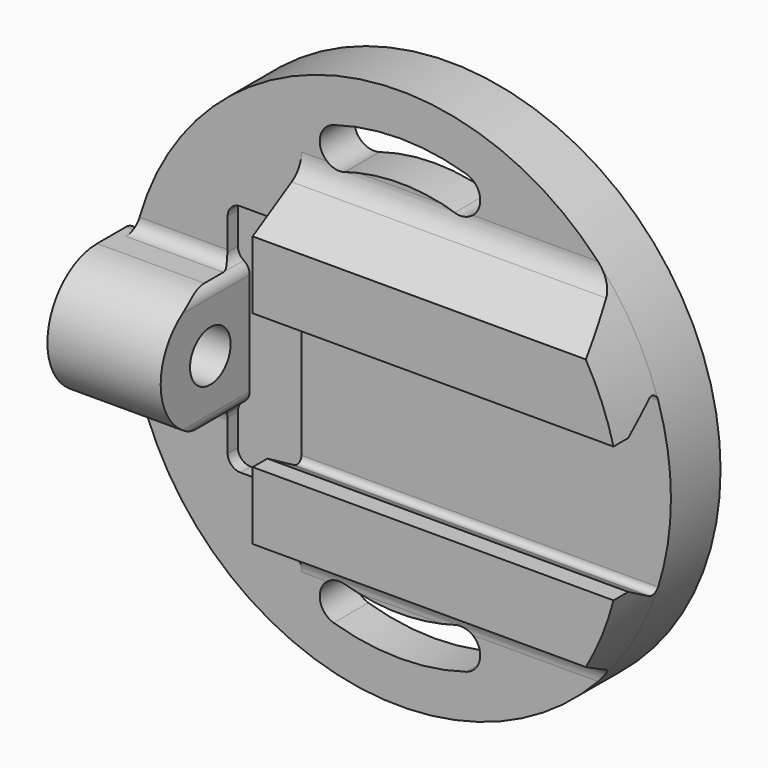
from build123d import *

# Parameters (mm, degrees)
F0_R           = 5.5025
F1_DEPTH       = 1.26
F2_R           = 5.03
F3_DEPTH       = 0.38
F4_R           = 2.75
F5_DEPTH       = 0.26
F7_DEPTH       = 7.5
F9_DEPTH       = 0.26
F10_R          = 0.26
F13_DEPTH      = 2.3
F14_R          = 0.765
F15_DEPTH      = 0.38
F16_R          = 0.515
F17_DEPTH      = 10.6835
F18_DEPTH      = 1.5
F19_F1_R       = 0.26
F19_F2_R       = 0.26
F21_DEPTH      = 15
F23_END_RADIUS = 5.5025
F23_REACH      = 10.1867902517
F25_DEPTH      = 10


# Not quite as in the source:
# - after a boolean that leaves OpenCascade's solid faulty, fix() repairs it


with BuildPart() as f1:
    # F0 (on Front) → F1 (new body)
    with BuildSketch(Plane.XZ):
        Circle(F0_R)
    extrude(amount=F1_DEPTH)

    # F2 (on face) → F3 (cut)
    with BuildSketch(Plane(origin=(0, 0, 0), x_dir=(-1, 0, 0), z_dir=(0, 1, 0))):
        Circle(F2_R)
    extrude(amount=-F3_DEPTH, mode=Mode.SUBTRACT)

    # F4 (on face) → F5 (cut)
    with BuildSketch(Plane(origin=(0, -0.38, 0), x_dir=(-1, 0, 0), z_dir=(0, 1, 0))):
        Circle(F4_R)
    extrude(amount=-F5_DEPTH, mode=Mode.SUBTRACT)

    # F6 (on face) → F7 (cut, symmetric)
    with BuildSketch(Plane.XZ.offset(1.26)):
        with BuildLine():
            ThreePointArc((-1.1142352941, 3.6852380804), (0, 3.85), (1.1142352941, 3.6852380804))
            ThreePointArc((1.1142352941, 3.6852380804), (1.6128818785, 3.952355253), (1.3457647059, 4.4510018374))
            ThreePointArc((1.3457647059, 4.4510018374), (0, 4.65), (-1.3457647059, 4.4510018374))
            ThreePointArc((-1.3457647059, 4.4510018374), (-1.6128818785, 3.952355253), (-1.1142352941, 3.6852380804))
        make_face()
        with BuildLine():
            ThreePointArc((1.1142352941, -3.6852380804), (0, -3.85), (-1.1142352941, -3.6852380804))
            ThreePointArc((-1.1142352941, -3.6852380804), (-1.6128818785, -3.952355253), (-1.3457647059, -4.4510018374))
            ThreePointArc((-1.3457647059, -4.4510018374), (0, -4.65), (1.3457647059, -4.4510018374))
            ThreePointArc((1.3457647059, -4.4510018374), (1.6128818785, -3.952355253), (1.1142352941, -3.6852380804))
        make_face()
    extrude(amount=F7_DEPTH, both=True, mode=Mode.SUBTRACT)

    # F8 (on face) → F9 (cut)
    with BuildSketch(Plane.XZ.offset(1.26)):
        with BuildLine():
            Line((-2, -2.38), (-2, 2.38))
            Line((-2, 2.38), (-3.5, 2.38))
            Line((-3.5, 2.38), (-3.5, 1.479089023))
            ThreePointArc((-3.5, 1.479089023), (-3.468035085, 1.354189063), (-3.38, 1.26))
            ThreePointArc((-3.38, 1.26), (-3.291964915, 1.165810937), (-3.26, 1.040910977))
            Line((-3.26, 1.040910977), (-3.26, -1.040910977))
            ThreePointArc((-3.26, -1.040910977), (-3.291964915, -1.165810937), (-3.38, -1.26))
            ThreePointArc((-3.38, -1.26), (-3.468035085, -1.354189063), (-3.5, -1.479089023))
            Line((-3.5, -1.479089023), (-3.5, -2.38))
            Line((-3.5, -2.38), (-2, -2.38))
        make_face()
    extrude(amount=-F9_DEPTH, mode=Mode.SUBTRACT)

    # F10
    f10_edges = [f1.edges().sort_by_distance(p)[0] for p in [
        (-2, -1.13, 2.38),
        (-3.5, -1.13, 2.38),
        (-3.5, -1.13, -2.38),
        (-2, -1.13, -2.38),
    ]]
    fillet(f10_edges, radius=F10_R)

    # F12 (on offset) → F13 (join, through all)
    with BuildSketch(Plane.YZ.offset(-5.56)):
        with BuildLine():
            Line((-1, -1.26), (-1, 1.26))
            Line((-1, 1.26), (-2, 1.26))
            ThreePointArc((-2, 1.26), (-3.26, 0), (-2, -1.26))
            Line((-2, -1.26), (-1, -1.26))
        make_face()
    extrude(amount=F13_DEPTH)

    # F14 (on face) → F15 (cut)
    with BuildSketch(Plane(origin=(-5.56, 0, 0), x_dir=(0, -1, 0), z_dir=(-1, 0, 0))):
        with Locations((2, 0)):
            Circle(F14_R)
    extrude(amount=-F15_DEPTH, mode=Mode.SUBTRACT)

    # F16 (on face) → F17 (cut, through all)
    with BuildSketch(Plane(origin=(-5.18, 0, 0), x_dir=(0, -1, 0), z_dir=(-1, 0, 0))):
        with Locations((2, 0)):
            Circle(F16_R)
    extrude(amount=-F17_DEPTH, mode=Mode.SUBTRACT)

    # F18 (cut): a face of the model
    f18_faces = [f1.faces().sort_by_distance(p)[0] for p in [
        (-2.6893148123, -1, 0),
    ]]
    extrude(f18_faces, amount=F18_DEPTH, mode=Mode.SUBTRACT)

    # F19: fillet of radius 0.26 on 4 edges, made by hand

    # F19_f1
    f19_f1_edges = [f1.edges().sort_by_distance(p)[0] for p in [
        (-5.4581479725, -1, 1.26),
        (-5.4581479725, -1, -1.26),
    ]]
    fillet(f19_f1_edges, radius=F19_F1_R)

    # F19_f2
    f19_f2_edges = [f1.edges().sort_by_distance(p)[0] for p in [
        (-4.3681479725, -1.26, 1.26),
        (-4.3681479725, -1.26, -1.26),
    ]]
    fillet(f19_f2_edges, radius=F19_F2_R)

    # F20 (on face) → F21 (cut)
    with BuildSketch(Plane.XZ.offset(1)):
        with BuildLine():
            ThreePointArc((-2.26, -2.38), (-2.0761522369, -2.3038477631), (-2, -2.12))
            Line((-2, -2.12), (-2, 2.12))
            ThreePointArc((-2, 2.12), (-2.0761522369, 2.3038477631), (-2.26, 2.38))
            Line((-2.26, 2.38), (-3.24, 2.38))
            ThreePointArc((-3.24, 2.38), (-3.4238477631, 2.3038477631), (-3.5, 2.12))
            Line((-3.5, 2.12), (-3.5, 1.479089023))
            ThreePointArc((-3.5, 1.479089023), (-3.468035085, 1.354189063), (-3.38, 1.26))
            ThreePointArc((-3.38, 1.26), (-3.2919649151, 1.165810937), (-3.2600000001, 1.0409109771))
            Line((-3.2600000001, 1.0409109771), (-3.2599999999, -1.0409109769))
            ThreePointArc((-3.2599999999, -1.0409109769), (-3.2919649149, -1.1658109369), (-3.38, -1.26))
            ThreePointArc((-3.38, -1.26), (-3.468035085, -1.354189063), (-3.5, -1.479089023))
            Line((-3.5, -1.479089023), (-3.5, -2.12))
            ThreePointArc((-3.5, -2.12), (-3.4238477631, -2.3038477631), (-3.24, -2.38))
            Line((-3.24, -2.38), (-2.26, -2.38))
        make_face()
    extrude(amount=F21_DEPTH, mode=Mode.SUBTRACT)

    f23_end = (Plane.ZX.offset(-0.76) * Cylinder(F23_END_RADIUS, 52.2556470224, mode=Mode.PRIVATE)).faces().sort_by_distance((-5.5025, -0.76, 0))[0]
    # F22 (on face) → F23 (join, up to the whole of a round face its end follows)
    with BuildSketch(Plane(origin=(-2, 0, 0), x_dir=(0, -1, 0), z_dir=(-1, 0, 0))):
        with BuildLine():
            Line((2.5, 2.75), (1.51, 3.3215767665))
            ThreePointArc((1.51, 3.3215767665), (1.3269872981, 3.5045894684), (1.26, 3.7545894684))
            Line((1.26, 3.7545894684), (1.26, 1.875))
            Line((1.26, 1.875), (1.26, 1.6671539031))
            ThreePointArc((1.26, 1.6671539031), (1.32, 1.7710769515), (1.44, 1.7710769515))
            Line((1.44, 1.7710769515), (2.1260254038, 1.375))
            Line((2.1260254038, 1.375), (2.5, 1.375))
            Line((2.5, 1.375), (2.5, 2.75))
        make_face()
        with BuildLine():
            ThreePointArc((1.26, -3.7545894684), (1.3269872981, -3.5045894684), (1.51, -3.3215767665))
            Line((1.51, -3.3215767665), (2.5, -2.75))
            Line((2.5, -2.75), (2.5, -1.375))
            Line((2.5, -1.375), (2.1260254038, -1.375))
            Line((2.1260254038, -1.375), (1.44, -1.7710769515))
            ThreePointArc((1.44, -1.7710769515), (1.32, -1.7710769515), (1.26, -1.6671539031))
            Line((1.26, -1.6671539031), (1.26, -1.875))
            Line((1.26, -1.875), (1.26, -3.7545894684))
        make_face()
    f23_long = extrude(amount=-F23_REACH, mode=Mode.PRIVATE)
    add(split(f23_long, bisect_by=f23_end, keep=Keep.BOTTOM, mode=Mode.PRIVATE))

    add(f1.part.fix(), mode=Mode.REPLACE)

    # F24 (on face) → F25 (cut)
    with BuildSketch(Plane(origin=(0, -0.38, 0), x_dir=(-1, 0, 0), z_dir=(0, 1, 0))):
        with BuildLine():
            ThreePointArc((-1.1142352941, -3.6852380804), (-1.6128818785, -3.952355253), (-1.3457647059, -4.4510018374))
            ThreePointArc((-1.3457647059, -4.4510018374), (0, -4.65), (1.3457647059, -4.4510018374))
            ThreePointArc((1.3457647059, -4.4510018374), (1.6128818785, -3.952355253), (1.1142352941, -3.6852380804))
            ThreePointArc((1.1142352941, -3.6852380804), (0, -3.85), (-1.1142352941, -3.6852380804))
        make_face()
        with BuildLine():
            ThreePointArc((-1.1142352941, 3.6852380804), (0, 3.85), (1.1142352941, 3.6852380804))
            ThreePointArc((1.1142352941, 3.6852380804), (1.6128818785, 3.952355253), (1.3457647059, 4.4510018374))
            ThreePointArc((1.3457647059, 4.4510018374), (0, 4.65), (-1.3457647059, 4.4510018374))
            ThreePointArc((-1.3457647059, 4.4510018374), (-1.6128818785, 3.952355253), (-1.1142352941, 3.6852380804))
        make_face()
    extrude(amount=-F25_DEPTH, mode=Mode.SUBTRACT)


solid = f1.part
